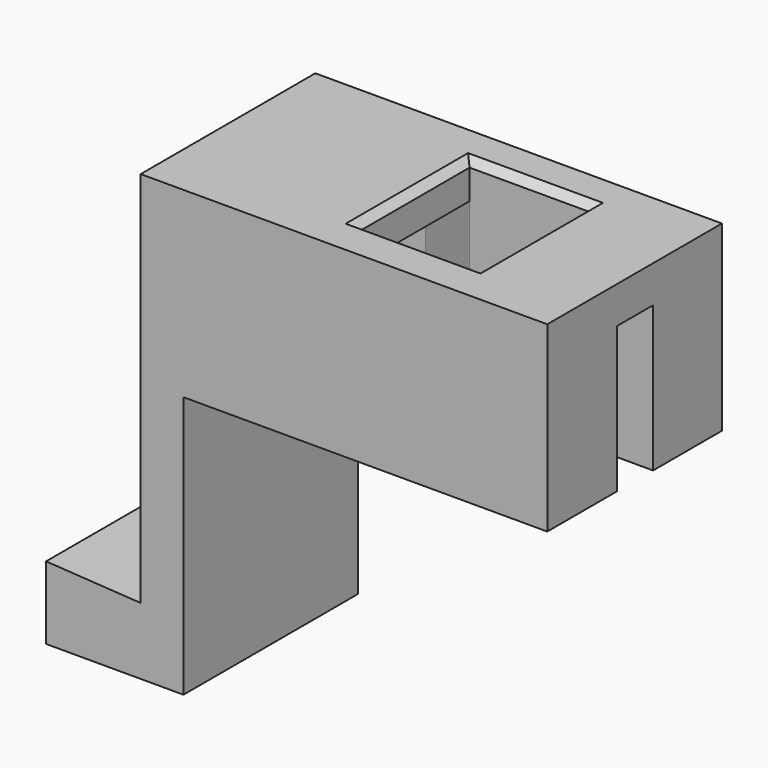
from build123d import *

# Parameters (mm, degrees)
F0_W     = 27.94
F0_H     = 15
F0_W_2   = 8.25
F0_H_2   = 9.5
F1_DEPTH = 2.54
F2_W     = 1.7651973286
F2_H     = 4.826
F2_W_2   = 1.3194764033
F3_DEPTH = 10
F4_W     = 2.94
F4_H     = 15
F5_DEPTH = 18
F6_W     = 15
F6_H     = 5
F7_DEPTH = 6.5
F9_DEPTH = 25.4
F10_SIZE = 0.508


# Not quite as in the source:
# - a feature names something its author has since deleted; it is built from what else it names


with BuildPart() as f1:
    # F0 (on Top) → F1 (new body)
    with BuildSketch(Plane.XY):
        with Locations((2.7402517554, 4.2405291848)):
            Rectangle(F0_W, F0_H)
        with Locations((5.5952517554, 4.3655291848)):
            Rectangle(F0_W_2, F0_H_2, mode=Mode.SUBTRACT)
    extrude(amount=F1_DEPTH)

    # F2 (on face) → F3 (join)
    with BuildSketch(Plane(origin=(0, 0, 0), x_dir=(1, 0, 0), z_dir=(0, 0, -1))):
        Polygon((-11.2297482446, -11.7405291848), (16.7102517554, -11.7405291848), (16.7102517554, -10.6549952576), (14.9450544268, -10.6549952576), (13.6255780235, -10.6549952576), (-2.7816970833, -10.6549952576), (-8.2897482446, -10.6549952576), (-11.2297482446, -10.6549952576), align=None)
        with Locations((15.8276530911, -8.2419952576)):
            Rectangle(F2_W, F2_H)
        with Locations((15.8276530911, -0.3159952576)):
            Rectangle(F2_W, F2_H)
        Polygon((-2.7816970833, -10.6549952576), (13.6255780235, -10.6549952576), (13.6255780235, -5.8289952576), (9.7202517554, -5.8289952576), (9.7202517554, -9.1155291848), (1.4702517554, -9.1155291848), align=None)
        Polygon((-8.2897482446, 3.2594708152), (-8.2897482446, 2.0970047424), (-2.7816970833, 2.0970047424), (13.6255780235, 2.0970047424), (14.9450544268, 2.0970047424), (16.7102517554, 2.0970047424), (16.7102517554, 3.2594708152), align=None)
        Polygon((13.6255780235, 2.0970047424), (-2.7816970833, 2.0970047424), (1.4702517554, 0.3844708152), (9.7202517554, 0.3844708152), (9.7202517554, -2.7289952576), (13.6255780235, -2.7289952576), align=None)
        with Locations((14.2853162251, -8.2419952576)):
            Rectangle(F2_W_2, F2_H)
        with Locations((14.2853162251, -0.3159952576)):
            Rectangle(F2_W_2, F2_H)
        Polygon((-11.2297482446, 3.2594708152), (-11.2297482446, -10.6549952576), (-8.2897482446, -10.6549952576), (-8.2897482446, 2.0970047424), (-8.2897482446, 3.2594708152), align=None)
    extrude(amount=F3_DEPTH)

    # F4 (on face) → F5 (join)
    with BuildSketch(Plane(origin=(0, 0, -10), x_dir=(1, 0, 0), z_dir=(0, 0, -1))):
        with Locations((-9.7597482446, -4.2405291848)):
            Rectangle(F4_W, F4_H)
    extrude(amount=F5_DEPTH)

    # F6 (on face) → F7 (join)
    with BuildSketch(Plane(origin=(-11.2297482446, 0, 0), x_dir=(0, -1, 0), z_dir=(-1, 0, 0))):
        with Locations((-4.2405291848, -25.5)):
            Rectangle(F6_W, F6_H)
    extrude(amount=F7_DEPTH)

    # F8 (on face) → F9 (cut)
    with BuildSketch(Plane.XZ.offset(3.2594708152)):
        Polygon((-11.2297482446, -23), (-17.7297482446, -23), (-11.2297482446, -23.4054420143), align=None)
    extrude(amount=-F9_DEPTH, mode=Mode.SUBTRACT)

    # F10
    f10_edges = [f1.edges().sort_by_distance(p)[0] for p in [
        (1.470252, 4.365529, 2.54),
        (5.595252, 9.115529, 2.54),
        (9.720252, 4.365529, 2.54),
        (5.595252, -0.384471, 2.54),
    ]]
    chamfer(f10_edges, length=F10_SIZE)


solid = f1.part
